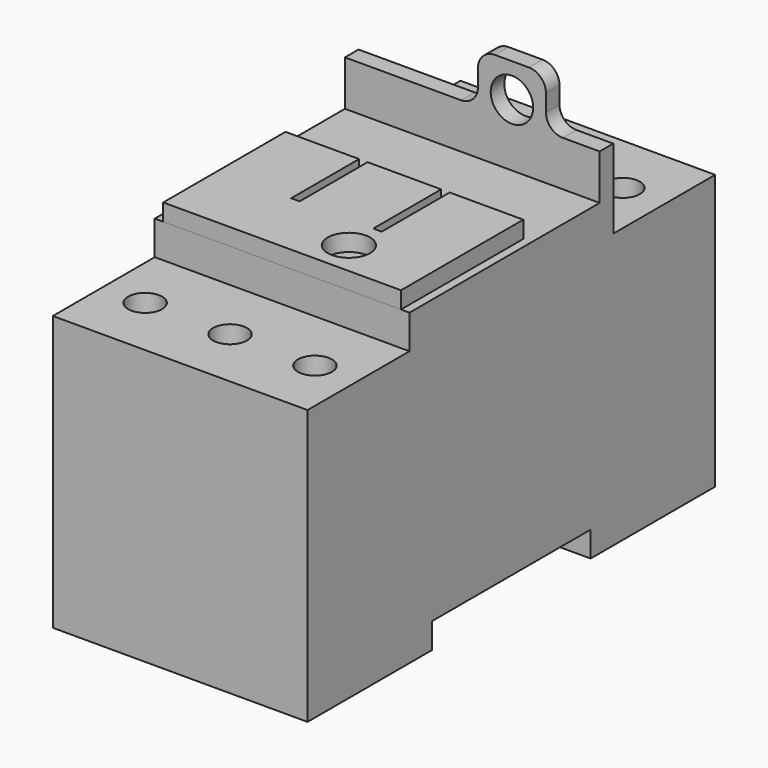
from build123d import *

# Parameters (mm, degrees)
F1_DEPTH = 22.5
F2_R     = 3.75
F3_DEPTH = 25
F5_DEPTH = 3
F6_R     = 3
F7_DEPTH = 25
F8_R     = 3.75
F9_DEPTH = 25


with BuildPart() as f1:
    # F0 (on Right) → F1 (new body, symmetric)
    with BuildSketch(Plane.YZ):
        Polygon((-45, 44), (-45, -4.5), (-17.5, -4.5), (-17.5, 0), (17.5, 0), (17.5, -4.5), (45, -4.5), (45, 44), (22.5, 44), (22.5, 67), (19.5, 67), (19.5, 50), (-22.5, 50), (-22.5, 44), align=None)
    extrude(amount=F1_DEPTH, both=True)

    # F2 (on face) → F3 (cut)
    with BuildSketch(Plane(origin=(0, 22.5, 0), x_dir=(-1, 0, 0), z_dir=(0, 1, 0))):
        with Locations((-7, 61)):
            Circle(F2_R)
        with BuildLine():
            Line((-13, 61), (-13, 64))
            ThreePointArc((-13, 64), (-12.1213203436, 66.1213203436), (-10, 67))
            Line((-10, 67), (-4, 67))
            ThreePointArc((-4, 67), (-1.8786796564, 66.1213203436), (-1, 64))
            Line((-1, 64), (-1, 61))
            ThreePointArc((-1, 61), (-0.1213203436, 58.8786796564), (2, 58))
            Line((2, 58), (22.5, 58))
            Line((22.5, 58), (37.2377703208, 58))
            Line((37.2377703208, 58), (37.2377703208, 73.085991472))
            Line((37.2377703208, 73.085991472), (-27.5872001182, 73.085991472))
            Line((-27.5872001182, 73.085991472), (-27.5872001182, 58))
            Line((-27.5872001182, 58), (-22.5, 58))
            Line((-22.5, 58), (-16, 58))
            ThreePointArc((-16, 58), (-13.8786796564, 58.8786796564), (-13, 61))
        make_face()
    extrude(amount=-F3_DEPTH, mode=Mode.SUBTRACT)

    # F6 (on face) → F7 (cut)
    with BuildSketch(Plane.XY.offset(44)):
        with Locations((15, -34)):
            Circle(F6_R)
        with Locations((-15, -34)):
            Circle(F6_R)
        with Locations((0, -34)):
            Circle(F6_R)
        with Locations((-15, 34)):
            Circle(F6_R)
        with Locations((0, 34)):
            Circle(F6_R)
        with Locations((15, 34)):
            Circle(F6_R)
    extrude(amount=-F7_DEPTH, mode=Mode.SUBTRACT)


with BuildPart() as f5:
    # F4 (on face) → F5 (new body)
    with BuildSketch(Plane.XY.offset(50)):
        Polygon((-21, -22.5), (21, -22.5), (21, 4.5), (8, 4.5), (8, -10.5), (6.5, -10.5), (6.5, 4.5), (-6.5, 4.5), (-6.5, -10.5), (-8, -10.5), (-8, 4.5), (-21, 4.5), align=None)
    extrude(amount=F5_DEPTH)

    # F8 (on face) → F9 (cut)
    with BuildSketch(Plane.XY.offset(53)):
        with Locations((7, -16.5)):
            Circle(F8_R)
    extrude(amount=-F9_DEPTH, mode=Mode.SUBTRACT)


solid = Compound([f1.part, f5.part])
